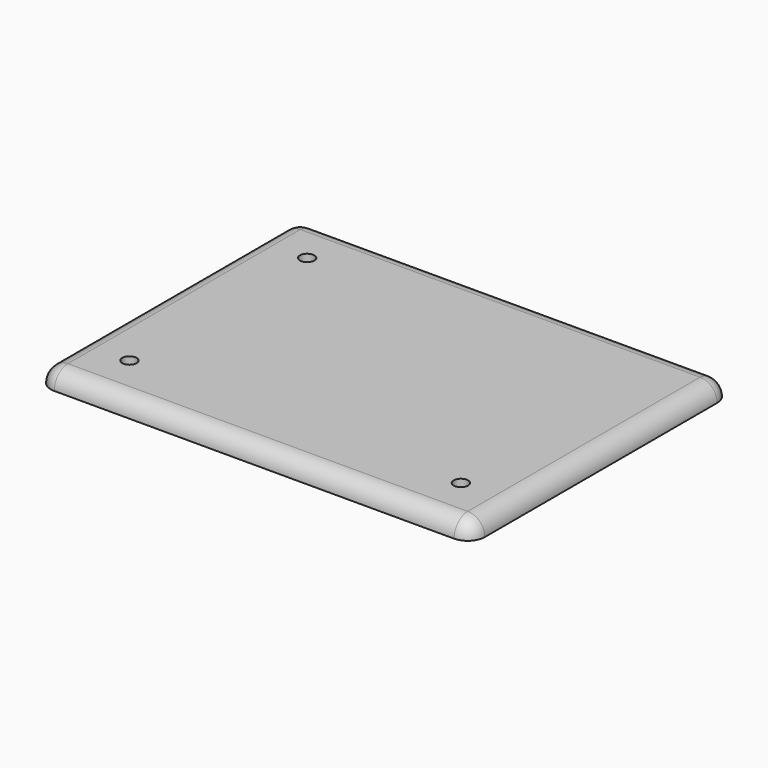
from build123d import *

# Parameters (mm, degrees)
F0_W     = 127
F0_H     = 95
F1_DEPTH = 5
F2_R     = 2.1
F3_DEPTH = 5.001
F4_R     = 4.99999


# Not quite as in the source:
# - a fillet or chamfer is up to 0.001 mm smaller than in the source, because OpenCascade refuses the exact size


with BuildPart() as f1:
    # F0 (on Top) → F1 (new body)
    with BuildSketch(Plane.XY):
        with Locations((1.5311012896, -0.0675843805)):
            Rectangle(F0_W, F0_H)
    extrude(amount=F1_DEPTH)

    # F2 (on face) → F3 (cut, through all)
    with BuildSketch(Plane.XY.offset(5)):
        with Locations((-46.9688987104, 32.4324156195)):
            Circle(F2_R)
        with Locations((-46.9688987104, -32.5675843805)):
            Circle(F2_R)
        with Locations((50.0311012896, -32.5675843805)):
            Circle(F2_R)
    extrude(amount=-F3_DEPTH, mode=Mode.SUBTRACT)

    # F4 (radius 5 in the source; OpenCascade refuses exactly that, so slightly less here)
    f4_edges = [f1.edges().sort_by_distance(p)[0] for p in [
        (1.531101, 47.432416, 5),
        (65.031101, -0.067584, 5),
        (-61.968899, -0.067584, 5),
        (1.531101, -47.567584, 5),
        (-61.968899, -47.567584, 2.5),
        (-61.968899, 47.432416, 2.5),
        (65.031101, 47.432416, 2.5),
        (65.031101, -47.567584, 2.5),
    ]]
    fillet(f4_edges, radius=F4_R)


solid = f1.part
